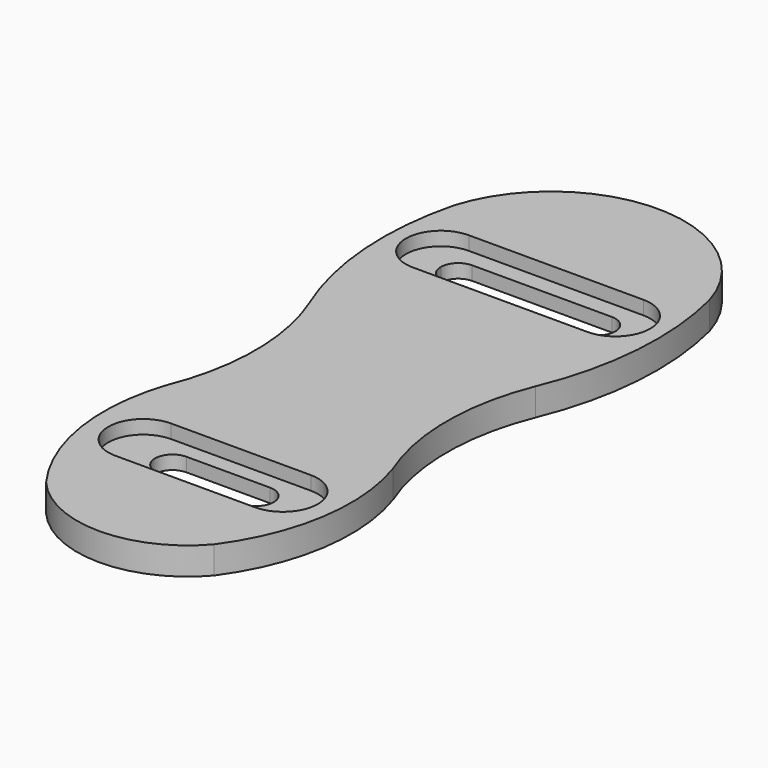
from build123d import *

# Parameters (mm, degrees)
F1_DEPTH = 10
F3_DEPTH = 5
F5_DEPTH = 25.4
F6_R     = 6.34999
F8_DEPTH = 5
F9_DEPTH = 25.4


# Not quite as in the source:
# - a fillet or chamfer is up to 0.001 mm smaller than in the source, because OpenCascade refuses the exact size


with BuildPart() as f1:
    # F0 (on Top) → F1 (new body)
    with BuildSketch(Plane.XY):
        with BuildLine():
            ThreePointArc((46.5285696909, 5.9739645023), (0, 40.5641849146), (-46.5285696909, 5.9739645023))
            ThreePointArc((-46.5285696909, 5.9739645023), (-49.6833366753, -30.6579453037), (-41.1537964933, -66.4224013325))
            ThreePointArc((-41.1537964933, -66.4224013325), (-34.8569562758, -98.8847496511), (-41.1537964933, -131.3470979697))
            ThreePointArc((-41.1537964933, -131.3470979697), (-44.1025989066, -166.693183735), (-30.5410850268, -199.467053752))
            ThreePointArc((-30.5410850268, -199.467053752), (0, -213.4927201844), (30.5410850268, -199.467053752))
            ThreePointArc((30.5410850268, -199.467053752), (44.1025989066, -166.693183735), (41.1537964933, -131.3470979697))
            ThreePointArc((41.1537964933, -131.3470979697), (34.8569562758, -98.8847496511), (41.1537964933, -66.4224013325))
            ThreePointArc((41.1537964933, -66.4224013325), (49.6833366753, -30.6579453037), (46.5285696909, 5.9739645023))
        make_face()
    extrude(amount=F1_DEPTH)

    # F2 (on face) → F3 (cut)
    with BuildSketch(Plane.XY.offset(10)):
        with BuildLine():
            Line((31.75, -5.715), (0, -5.715))
            Line((0, -5.715), (0, -18.415))
            Line((0, -18.415), (-19.05, -18.415))
            ThreePointArc((-19.05, -18.415), (-22.7697438789, -27.3952561211), (-31.75, -31.115))
            Line((-31.75, -31.115), (31.75, -31.115))
            ThreePointArc((31.75, -31.115), (19.05, -18.415), (31.75, -5.715))
        make_face()
        with BuildLine():
            Line((0, -18.415), (0, -5.715))
            Line((0, -5.715), (-31.75, -5.715))
            ThreePointArc((-31.75, -5.715), (-22.7697438789, -9.4347438789), (-19.05, -18.415))
            Line((-19.05, -18.415), (0, -18.415))
        make_face()
        with BuildLine():
            ThreePointArc((-19.05, -18.415), (-22.7697438789, -9.4347438789), (-31.75, -5.715))
            ThreePointArc((-31.75, -5.715), (-44.45, -18.415), (-31.75, -31.115))
            ThreePointArc((-31.75, -31.115), (-22.7697438789, -27.3952561211), (-19.05, -18.415))
        make_face()
        with BuildLine():
            ThreePointArc((44.45, -18.415), (40.7302561211, -9.4347438789), (31.75, -5.715))
            ThreePointArc((31.75, -5.715), (19.05, -18.415), (31.75, -31.115))
            ThreePointArc((31.75, -31.115), (40.7302561211, -27.3952561211), (44.45, -18.415))
        make_face()
    extrude(amount=-F3_DEPTH, mode=Mode.SUBTRACT)

    # F4 (on face) → F5 (cut)
    with BuildSketch(Plane.XY.offset(5)):
        Polygon((-31.75, -12.065), (-31.75, -18.415), (-31.75, -24.765), (31.75, -24.765), (31.75, -12.065), align=None)
    extrude(amount=-F5_DEPTH, mode=Mode.SUBTRACT)

    # F6 (radius 6.35 in the source; OpenCascade refuses exactly that, so slightly less here)
    f6_edges = [f1.edges().sort_by_distance(p)[0] for p in [
        (-31.75, -12.065, 2.5),
        (-31.75, -24.765, 2.5),
        (31.75, -12.065, 2.5),
        (31.75, -24.765, 2.5),
    ]]
    fillet(f6_edges, radius=F6_R)

    # F7 (on face) → F8 (cut)
    with BuildSketch(Plane.XY.offset(10)):
        with BuildLine():
            Line((25.4, -148.9900371552), (-25.4, -148.9900371552))
            ThreePointArc((-25.4, -148.9900371552), (-38.1, -161.6900371552), (-25.4, -174.3900371552))
            Line((-25.4, -174.3900371552), (25.4, -174.3900371552))
            ThreePointArc((25.4, -174.3900371552), (38.1, -161.6900371552), (25.4, -148.9900371552))
        make_face()
        with BuildLine():
            ThreePointArc((-15.24, -167.4590520005), (-21.59, -161.1090520005), (-15.24, -154.7590520005))
            Line((-15.24, -154.7590520005), (15.24, -154.7590520005))
            ThreePointArc((15.24, -154.7590520005), (21.59, -161.1090520005), (15.24, -167.4590520005))
            Line((15.24, -167.4590520005), (-15.24, -167.4590520005))
        make_face(mode=Mode.SUBTRACT)
    extrude(amount=-F8_DEPTH, mode=Mode.SUBTRACT)

    # F9 (cut): a face of the model
    f9_faces = [f1.faces().sort_by_distance(p)[0] for p in [
        (0, -161.1090520005, 10),
    ]]
    extrude(f9_faces, amount=-F9_DEPTH, mode=Mode.SUBTRACT)


solid = f1.part
